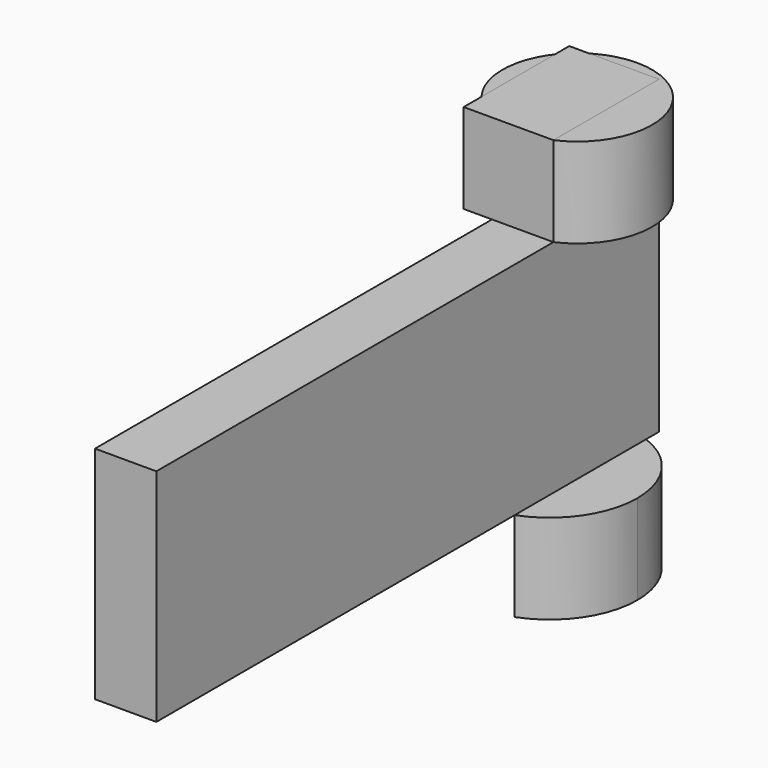
from build123d import *

# Parameters (mm, degrees)
F0_W     = 17.3768736422
F0_H     = 62.4421741813
F1_DEPTH = 127
F2_DEPTH = 50.8
F4_DEPTH = 25.4
F6_DEPTH = 25.4
F7_W     = 8.6884368211
F7_H     = 31.1260204762
F8_DEPTH = 25.4
F9_DEPTH = 25.4


with BuildPart() as f1:
    # F0 (on Front) → F1 (new body)
    with BuildSketch(Plane.XZ):
        with Locations((-46.5929340571, 16.8040106073)):
            Rectangle(F0_W, F0_H)
    extrude(amount=F1_DEPTH)

    # F2 (add): a face of the model
    f2_faces = [f1.faces().sort_by_distance(p)[0] for p in [
        (-46.5929340571, -127, 16.8040106073),
    ]]
    extrude(f2_faces, amount=F2_DEPTH)


with BuildPart() as f4:
    # F3 (on face) → F4 (new body)
    with BuildSketch(Plane.XY.offset(48.025097698)):
        with BuildLine():
            ThreePointArc((-37.904497236, -37.3494494503), (-28.8159794009, -29.5392090488), (-25.4241662195, -18.0458799005))
            ThreePointArc((-25.4241662195, -18.0458799005), (-58.0862632055, -0.2689252442), (-55.2813708782, -37.3494494503))
            Line((-55.2813708782, -37.3494494503), (-55.2813708782, 0))
            Line((-55.2813708782, 0), (-37.904497236, 0))
            Line((-37.904497236, 0), (-37.904497236, -37.3494494503))
        make_face()
    extrude(amount=F4_DEPTH)


with BuildPart() as f6:
    # F5 (on face) → F6 (new body)
    with BuildSketch(Plane(origin=(0, 0, -14.4170764834), x_dir=(1, 0, 0), z_dir=(0, 0, -1))):
        with BuildLine():
            ThreePointArc((-37.904497236, 4.5781515434), (-26.2133427827, 13.6756799094), (-21.7906919048, 27.8138648719))
            ThreePointArc((-21.7906919048, 27.8138648719), (-26.2133427827, 41.9520498344), (-37.904497236, 51.0495782003))
            Line((-37.904497236, 51.0495782003), (-37.904497236, 4.5781515434))
        make_face()
    extrude(amount=F6_DEPTH)


with BuildPart() as f8:
    # F7 (on face) → F8 (new body)
    with BuildSketch(Plane.XY.offset(48.025097698)):
        with Locations((-50.9371524677, -15.5630102381)):
            Rectangle(F7_W, F7_H)
    extrude(amount=F8_DEPTH)


with BuildPart() as f9:
    # F9 (new): a face of the model
    f9_faces = [f4.part.faces().sort_by_distance(p)[0] for p in [
        (-37.904497236, -18.6747247252, 60.725097698),
    ]]
    extrude(f9_faces, amount=F9_DEPTH)


solid = Compound([f1.part, f4.part, f6.part, f8.part, f9.part])
